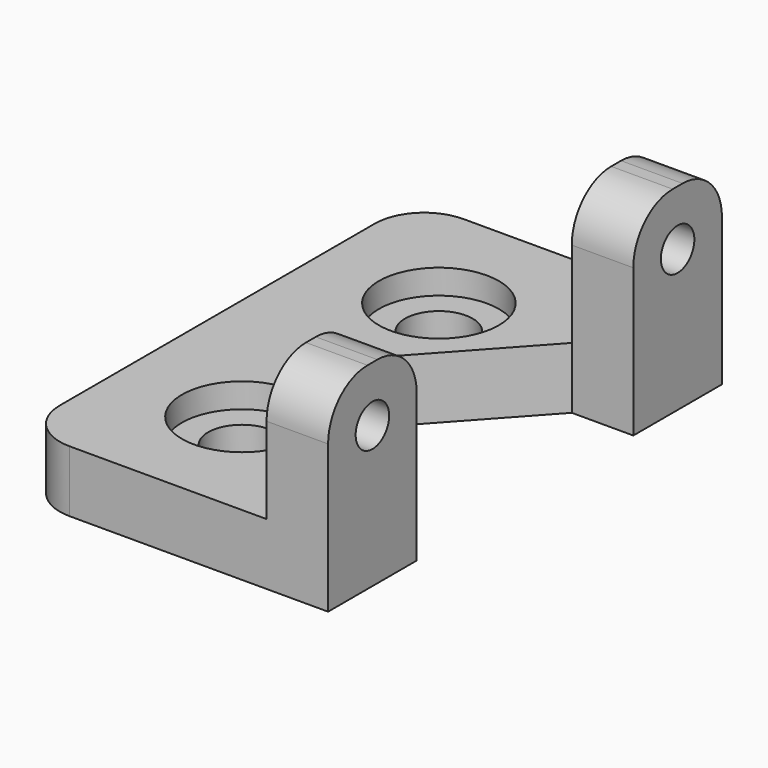
from build123d import *

# Parameters (mm, degrees)
F0_W           = 11
F0_H           = 9
F0_R           = 1.7
F1_DEPTH       = 5
F2_DEPTH       = 25
F4_D           = 5.5
F4_CBORE_D     = 9.75
F4_CBORE_DEPTH = 2
F5_DEPTH       = 5.001
F6_R           = 4
F7_ANGLE       = 90


# Not quite as in the source:
# - a feature names something its author has since deleted; it is built from what else it names


with BuildPart() as f1:
    # F0 (on Top) → F1 (new body)
    with BuildSketch(Plane.XY):
        with Locations((-48.0971363783, -35.5)):
            Rectangle(F0_W, F0_H)
        with Locations((-47.0971363783, -35.5)):
            Circle(F0_R, mode=Mode.SUBTRACT)
    extrude(amount=F1_DEPTH)



with BuildPart() as f1b:
    # F0 (on Top) → F1, piece 2 (new body)
    with BuildSketch(Plane.XY):
        with Locations((-48.0971363783, -4.5)):
            Rectangle(F0_W, F0_H)
        with Locations((-47.0971363783, -4.5)):
            Circle(F0_R, mode=Mode.SUBTRACT)
    extrude(amount=F1_DEPTH)


with BuildPart() as f1_1:
    add(f1.part)

    add(f1b.part)  # F2 merges F1b
    # F0 (on Top) → F2 (join)
    with BuildSketch(Plane.XY):
        Polygon((-58.5971363783, -40), (-53.5971363783, -40), (-53.5971363783, -31), (-53.5971363783, -9), (-53.5971363783, 0), (-58.5971363783, 0), align=None)
    extrude(amount=F2_DEPTH)

    # F4 (through all)
    with Locations(Plane.YZ.offset(-53.5971363783)):
        with Locations((-10, 15), (-30, 15)):
            CounterBoreHole(F4_D / 2, F4_CBORE_D / 2, F4_CBORE_DEPTH)

    # F3 (on face) → F5 (cut, through all)
    with BuildSketch(Plane.YZ.offset(-53.5971363783)):
        Polygon((-20, 15), (-31, 5), (-31, 0), (-9, 0), (-9, 5), align=None)
    extrude(amount=-F5_DEPTH, mode=Mode.SUBTRACT)

    # F6
    f6_edges = [f1_1.edges().sort_by_distance(p)[0] for p in [
        (-42.597136, 0, 2.5),
        (-42.597136, -40, 2.5),
        (-56.097136, -40, 25),
        (-56.097136, 0, 25),
        (-42.597136, -9, 2.5),
        (-42.597136, -31, 2.5),
        (-56.097136, -20, 15),
    ]]
    fillet(f6_edges, radius=F6_R)


with BuildPart() as f1_2:
    # F7: moved
    add(f1_1.part.rotate(Axis((-58.5971363783, -20, 0), (0, -1, 0)), F7_ANGLE))


solid = f1_2.part
